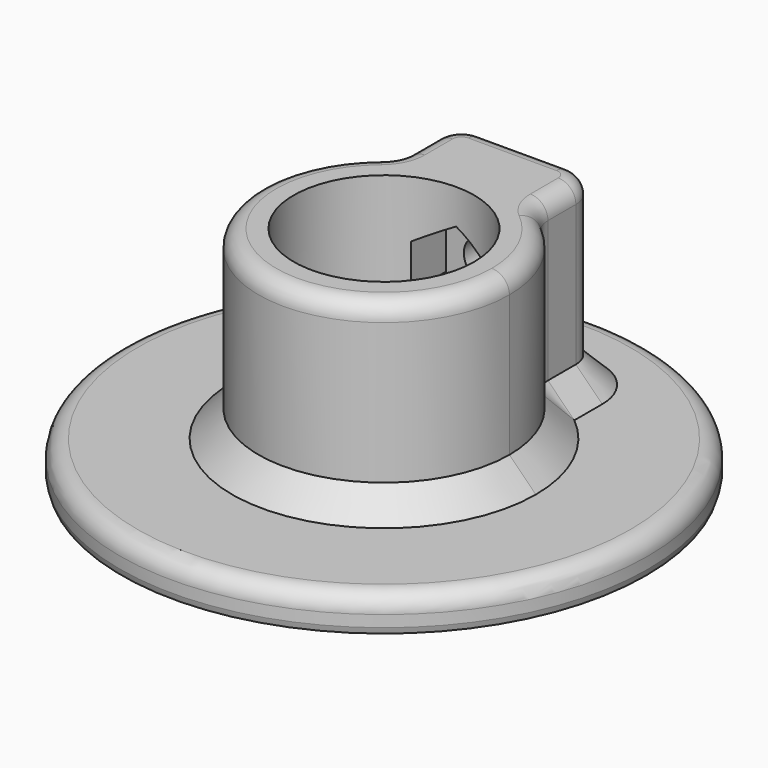
from build123d import *

# Parameters (mm, degrees)
F0_R     = 30
F0_R_2   = 10.25
F1_DEPTH = 4
F2_DEPTH = 25
F3_R     = 3
F4_SIZE  = 2.99999
F6_SIZE2 = 0.7
F6_SIZE  = 0.2
F7_START = -6
F7_DEPTH = 19
F8_D     = 4.65
F8_DEPTH = 8
F8_TIP   = 1.3970009392
F9_R     = 2


# Not quite as in the source:
# - a fillet or chamfer is up to 0.001 mm smaller than in the source, because OpenCascade refuses the exact size


with BuildPart() as f1:
    # F0 (on Top) → F1 (new body)
    with BuildSketch(Plane.XY):
        Circle(F0_R)
        with BuildLine():
            ThreePointArc((8, 11.7924764151), (12.5909193469, 6.6731739075), (14.25, 0))
            ThreePointArc((14.25, 0), (-6.6731739075, -12.5909193469), (-8, 11.7924764151))
            Line((-8, 11.7924764151), (-8, 20.25))
            Line((-8, 20.25), (8, 20.25))
            Line((8, 20.25), (8, 11.7924764151))
        make_face(mode=Mode.SUBTRACT)
        with BuildLine():
            ThreePointArc((-8, 11.7924764151), (0, 14.25), (8, 11.7924764151))
            Line((8, 11.7924764151), (8, 20.25))
            Line((8, 20.25), (-8, 20.25))
            Line((-8, 20.25), (-8, 11.7924764151))
        make_face()
        with BuildLine():
            ThreePointArc((-8, 11.7924764151), (-6.6731739075, -12.5909193469), (14.25, 0))
            ThreePointArc((14.25, 0), (12.5909193469, 6.6731739075), (8, 11.7924764151))
            ThreePointArc((8, 11.7924764151), (0, 14.25), (-8, 11.7924764151))
        make_face()
        Circle(F0_R_2, mode=Mode.SUBTRACT)
    extrude(amount=F1_DEPTH)

    # F0 (on Top) → F2 (join)
    with BuildSketch(Plane.XY):
        with BuildLine():
            ThreePointArc((-8, 11.7924764151), (0, 14.25), (8, 11.7924764151))
            Line((8, 11.7924764151), (8, 20.25))
            Line((8, 20.25), (-8, 20.25))
            Line((-8, 20.25), (-8, 11.7924764151))
        make_face()
        with BuildLine():
            ThreePointArc((-8, 11.7924764151), (-6.6731739075, -12.5909193469), (14.25, 0))
            ThreePointArc((14.25, 0), (12.5909193469, 6.6731739075), (8, 11.7924764151))
            ThreePointArc((8, 11.7924764151), (0, 14.25), (-8, 11.7924764151))
        make_face()
        Circle(F0_R_2, mode=Mode.SUBTRACT)
    extrude(amount=F2_DEPTH)

    # F3
    f3_edges = [f1.edges().sort_by_distance(p)[0] for p in [
        (-8, 11.792476, 14.5),
        (8, 11.792476, 14.5),
        (8, 20.25, 14.5),
        (-8, 20.25, 14.5),
    ]]
    fillet(f3_edges, radius=F3_R)

    # F4 (size 3 in the source; OpenCascade refuses exactly that, so slightly less here)
    f4_edges = [f1.edges().sort_by_distance(p)[0] for p in [
        (0, -14.25, 4),
        (-8, 15.268841, 4),
        (8, 15.268841, 4),
    ]]
    chamfer(f4_edges, length=F4_SIZE)

    # F6
    f6_edges = [f1.edges().sort_by_distance(p)[0] for p in [
        (-10.25, 0, 0),
        (-30, 0, 0),
    ]]
    f6_side = f1.faces().sort_by_distance((-29.151472, 0, 0))[0]
    chamfer(f6_edges, length=F6_SIZE, length2=F6_SIZE2, reference=f6_side)

    # F5 (on face) → F7 (cut)
    with BuildSketch(Plane(origin=(0, 20.25, 0), x_dir=(-1, 0, 0), z_dir=(0, 1, 0)).offset(F7_START)):
        Polygon((-4.36, 18.5172471737), (-4.36, 13.4827528263), (0, 10.9655056527), (4.36, 13.4827528263), (4.36, 18.5172471737), (0, 21.0344943473), align=None)
    extrude(amount=-F7_DEPTH, mode=Mode.SUBTRACT)

    # F8
    with Locations(Plane(origin=(0, 20.25, 0), x_dir=(-1, 0, 0), z_dir=(0, 1, 0))):
        with Locations((0, 16)):
            Hole(F8_D / 2, depth=F8_DEPTH)
            with Locations((0, 0, -(F8_DEPTH + F8_TIP / 2))):  # 118° drill point
                Cone(0, F8_D / 2, F8_TIP, mode=Mode.SUBTRACT)

    # F9
    f9_edges = [f1.edges().sort_by_distance(p)[0] for p in [
        (-30, 0, 4),
        (0, -14.25, 25),
    ]]
    fillet(f9_edges, radius=F9_R)


solid = f1.part
